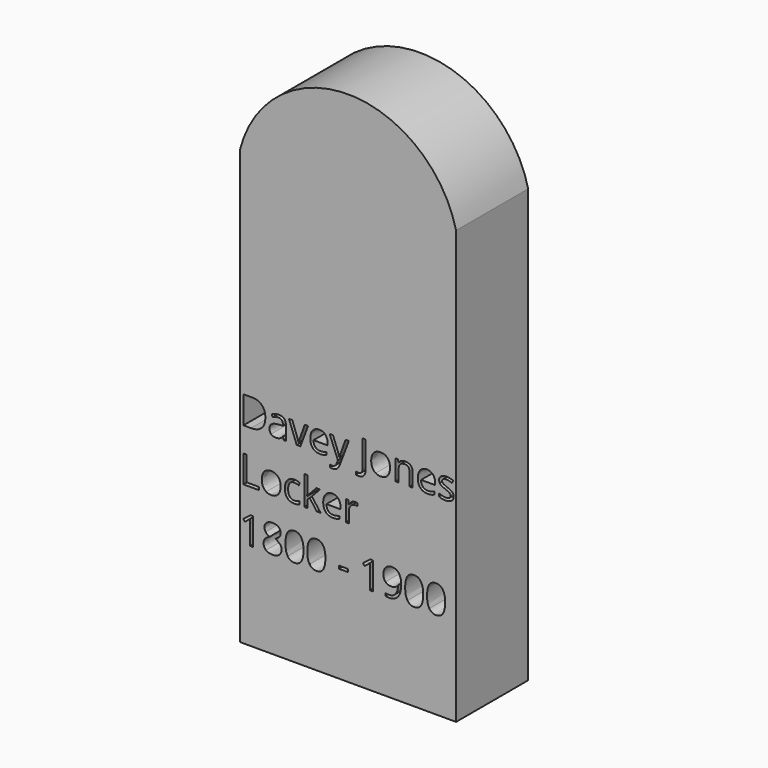
from build123d import *

# Parameters (mm, degrees)
F0_W     = 12.9239648405
F0_H     = 4.0018795953
F1_DEPTH = 127


with BuildPart() as f1:
    # F0 (on Front) → F1 (new body)
    with BuildSketch(Plane.XZ):
        with BuildLine():
            Line((-39.4293889403, 317.6073561937), (-39.4293889403, -291.9926438063))
            Line((-39.4293889403, -291.9926438063), (265.3706110597, -291.9926438063))
            Line((265.3706110597, -291.9926438063), (265.3706110597, 317.6073561937))
            ThreePointArc((265.3706110597, 317.6073561937), (112.9706110597, 436.9978931719), (-39.4293889403, 317.6073561937))
        make_face()
        with BuildLine():
            Line((-20.6079173278, -129.7050005513), (-20.6079173278, -168.1988697536))
            Line((-20.6079173278, -168.1988697536), (-24.870972223, -168.1988697536))
            Line((-24.870972223, -168.1988697536), (-24.870972223, -140.7670382538))
            add(Edge.make_bspline(
                [(-24.870972223, -140.7670382538), (-24.870972223, -137.3380593163), (-24.6603469811, -134.2882058142)],
                knots=[0, 0, 0, 1, 1, 1], degree=2))
            add(Edge.make_bspline(
                [(-24.6603469811, -134.2882058142), (-25.20797261, -134.8442564527), (-25.8946108984, -135.4466446444)],
                knots=[0, 0, 0, 1, 1, 1], degree=2))
            add(Edge.make_bspline(
                [(-25.8946108984, -135.4466446444), (-26.5812491869, -136.0490328361), (-32.1586055913, -140.5816880409)],
                knots=[0, 0, 0, 1, 1, 1], degree=2))
            Line((-32.1586055913, -140.5816880409), (-34.4754832518, -137.5823845969))
            Line((-34.4754832518, -137.5823845969), (-24.2896465555, -129.7050005513))
            Line((-24.2896465555, -129.7050005513), (-20.6079173278, -129.7050005513))
        make_face(mode=Mode.SUBTRACT)
        with BuildLine():
            add(Edge.make_bspline(
                [(-1.5084203959, -131.6427527764), (1.5835581546, -129.1573749225), (6.773364114, -129.1573749225)],
                knots=[0, 0, 0, 1, 1, 1], degree=2))
            add(Edge.make_bspline(
                [(6.773364114, -129.1573749225), (12.0389951605, -129.1573749225), (15.1183361965, -131.6048402329)],
                knots=[0, 0, 0, 1, 1, 1], degree=2))
            add(Edge.make_bspline(
                [(15.1183361965, -131.6048402329), (18.1976772325, -134.0523055433), (18.1976772325, -138.3659104966)],
                knots=[0, 0, 0, 1, 1, 1], degree=2))
            add(Edge.make_bspline(
                [(18.1976772325, -138.3659104966), (18.1976772325, -141.2135637665), (16.4368502105, -143.555716456)],
                knots=[0, 0, 0, 1, 1, 1], degree=2))
            add(Edge.make_bspline(
                [(16.4368502105, -143.555716456), (14.6760231886, -145.8978691455), (10.8005187384, -147.8187713512)],
                knots=[0, 0, 0, 1, 1, 1], degree=2))
            add(Edge.make_bspline(
                [(10.8005187384, -147.8187713512), (15.4848241173, -150.0598239246), (17.460488886, -152.5199267496)],
                knots=[0, 0, 0, 1, 1, 1], degree=2))
            add(Edge.make_bspline(
                [(17.460488886, -152.5199267496), (19.4361536546, -154.9800295745), (19.4361536546, -158.2236582991)],
                knots=[0, 0, 0, 1, 1, 1], degree=2))
            add(Edge.make_bspline(
                [(19.4361536546, -158.2236582991), (19.4361536546, -163.0090637942), (16.0914248139, -165.8693545786)],
                knots=[0, 0, 0, 1, 1, 1], degree=2))
            add(Edge.make_bspline(
                [(16.0914248139, -165.8693545786), (12.7466959731, -168.7296453631), (6.9334392978, -168.7296453631)],
                knots=[0, 0, 0, 1, 1, 1], degree=2))
            add(Edge.make_bspline(
                [(6.9334392978, -168.7296453631), (0.7747572258, -168.7296453631), (-2.5446965859, -166.0294297624)],
                knots=[0, 0, 0, 1, 1, 1], degree=2))
            add(Edge.make_bspline(
                [(-2.5446965859, -166.0294297624), (-5.8641503976, -163.3292141618), (-5.8641503976, -158.3753084732)],
                knots=[0, 0, 0, 1, 1, 1], degree=2))
            add(Edge.make_bspline(
                [(-5.8641503976, -158.3753084732), (-5.8641503976, -151.7701008885), (2.1901588511, -148.0799466511)],
                knots=[0, 0, 0, 1, 1, 1], degree=2))
            add(Edge.make_bspline(
                [(2.1901588511, -148.0799466511), (-1.4410203185, -146.0326693003), (-3.0207096325, -143.6483915624)],
                knots=[0, 0, 0, 1, 1, 1], degree=2))
            add(Edge.make_bspline(
                [(-3.0207096325, -143.6483915624), (-4.6003989464, -141.2641138246), (-4.6003989464, -138.3153604385)],
                knots=[0, 0, 0, 1, 1, 1], degree=2))
            add(Edge.make_bspline(
                [(-4.6003989464, -138.3153604385), (-4.6003989464, -134.1281306304), (-1.5084203959, -131.6427527764)],
                knots=[0, 0, 0, 1, 1, 1], degree=2))
        make_face(mode=Mode.SUBTRACT)
        with BuildLine():
            add(Edge.make_bspline(
                [(47.1207354447, -134.1828931932), (50.372789179, -139.2673865317), (50.372789179, -148.8971725896)],
                knots=[0, 0, 0, 1, 1, 1], degree=2))
            add(Edge.make_bspline(
                [(50.372789179, -148.8971725896), (50.372789179, -158.8808090537), (47.2260480656, -163.8052272084)],
                knots=[0, 0, 0, 1, 1, 1], degree=2))
            add(Edge.make_bspline(
                [(47.2260480656, -163.8052272084), (44.0793069522, -168.7296453631), (37.6004745126, -168.7296453631)],
                knots=[0, 0, 0, 1, 1, 1], degree=2))
            add(Edge.make_bspline(
                [(37.6004745126, -168.7296453631), (31.3912423826, -168.7296453631), (28.1518261628, -163.687277073)],
                knots=[0, 0, 0, 1, 1, 1], degree=2))
            add(Edge.make_bspline(
                [(28.1518261628, -163.687277073), (24.912409943, -158.6449087828), (24.912409943, -148.8971725896)],
                knots=[0, 0, 0, 1, 1, 1], degree=2))
            add(Edge.make_bspline(
                [(24.912409943, -148.8971725896), (24.912409943, -138.846136048), (28.0465135418, -133.9722679514)],
                knots=[0, 0, 0, 1, 1, 1], degree=2))
            add(Edge.make_bspline(
                [(28.0465135418, -133.9722679514), (31.1806171407, -129.0983998548), (37.6004745126, -129.0983998548)],
                knots=[0, 0, 0, 1, 1, 1], degree=2))
            add(Edge.make_bspline(
                [(37.6004745126, -129.0983998548), (43.8686817103, -129.0983998548), (47.1207354447, -134.1828931932)],
                knots=[0, 0, 0, 1, 1, 1], degree=2))
        make_face(mode=Mode.SUBTRACT)
        with BuildLine():
            add(Edge.make_bspline(
                [(77.9478458432, -134.1828931932), (81.1998995775, -139.2673865317), (81.1998995775, -148.8971725896)],
                knots=[0, 0, 0, 1, 1, 1], degree=2))
            add(Edge.make_bspline(
                [(81.1998995775, -148.8971725896), (81.1998995775, -158.8808090537), (78.0531584642, -163.8052272084)],
                knots=[0, 0, 0, 1, 1, 1], degree=2))
            add(Edge.make_bspline(
                [(78.0531584642, -163.8052272084), (74.9064173508, -168.7296453631), (68.4275849112, -168.7296453631)],
                knots=[0, 0, 0, 1, 1, 1], degree=2))
            add(Edge.make_bspline(
                [(68.4275849112, -168.7296453631), (62.2183527812, -168.7296453631), (58.9789365614, -163.687277073)],
                knots=[0, 0, 0, 1, 1, 1], degree=2))
            add(Edge.make_bspline(
                [(58.9789365614, -163.687277073), (55.7395203415, -158.6449087828), (55.7395203415, -148.8971725896)],
                knots=[0, 0, 0, 1, 1, 1], degree=2))
            add(Edge.make_bspline(
                [(55.7395203415, -148.8971725896), (55.7395203415, -138.846136048), (58.8736239404, -133.9722679514)],
                knots=[0, 0, 0, 1, 1, 1], degree=2))
            add(Edge.make_bspline(
                [(58.8736239404, -133.9722679514), (62.0077275393, -129.0983998548), (68.4275849112, -129.0983998548)],
                knots=[0, 0, 0, 1, 1, 1], degree=2))
            add(Edge.make_bspline(
                [(68.4275849112, -129.0983998548), (74.6957921089, -129.0983998548), (77.9478458432, -134.1828931932)],
                knots=[0, 0, 0, 1, 1, 1], degree=2))
        make_face(mode=Mode.SUBTRACT)
        with Locations((106.5676037071, -153.7457656572)):
            Rectangle(F0_W, F0_H, mode=Mode.SUBTRACT)
        Polygon((-12.6799832242, -94.8675855477), (-34.1384828648, -94.8675855477), (-34.1384828648, -56.3737163454), (-29.6648027277, -56.3737163454), (-29.6648027277, -90.8151558943), (-12.6799832242, -90.8151558943), align=None, mode=Mode.SUBTRACT)
        with BuildLine():
            add(Edge.make_bspline(
                [(14.5285855193, -69.5125189326), (18.0965771164, -73.5438860618), (18.0965771164, -80.4102689465)],
                knots=[0, 0, 0, 1, 1, 1], degree=2))
            add(Edge.make_bspline(
                [(18.0965771164, -80.4102689465), (18.0965771164, -87.4704270536), (14.5454355386, -91.4343941054)],
                knots=[0, 0, 0, 1, 1, 1], degree=2))
            add(Edge.make_bspline(
                [(14.5454355386, -91.4343941054), (10.9942939609, -95.3983611572), (4.7260867631, -95.3983611572)],
                knots=[0, 0, 0, 1, 1, 1], degree=2))
            add(Edge.make_bspline(
                [(4.7260867631, -95.3983611572), (0.8505823129, -95.3983611572), (-2.1487211312, -93.5785590675)],
                knots=[0, 0, 0, 1, 1, 1], degree=2))
            add(Edge.make_bspline(
                [(-2.1487211312, -93.5785590675), (-5.1480245753, -91.7587569779), (-6.7824764521, -88.3634780791)],
                knots=[0, 0, 0, 1, 1, 1], degree=2))
            add(Edge.make_bspline(
                [(-6.7824764521, -88.3634780791), (-8.4169283289, -84.9681991803), (-8.4169283289, -80.4102689465)],
                knots=[0, 0, 0, 1, 1, 1], degree=2))
            add(Edge.make_bspline(
                [(-8.4169283289, -80.4102689465), (-8.4169283289, -73.358535849), (-4.8868492753, -69.4198438262)],
                knots=[0, 0, 0, 1, 1, 1], degree=2))
            add(Edge.make_bspline(
                [(-4.8868492753, -69.4198438262), (-1.3567702218, -65.4811518035), (4.911436976, -65.4811518035)],
                knots=[0, 0, 0, 1, 1, 1], degree=2))
            add(Edge.make_bspline(
                [(4.911436976, -65.4811518035), (10.9605939222, -65.4811518035), (14.5285855193, -69.5125189326)],
                knots=[0, 0, 0, 1, 1, 1], degree=2))
        make_face(mode=Mode.SUBTRACT)
        with BuildLine():
            add(Edge.make_bspline(
                [(44.5848075327, -93.8902844255), (41.6950292143, -95.3983611572), (37.2971741643, -95.3983611572)],
                knots=[0, 0, 0, 1, 1, 1], degree=2))
            add(Edge.make_bspline(
                [(37.2971741643, -95.3983611572), (31.0289669666, -95.3983611572), (27.5915630194, -91.5397067263)],
                knots=[0, 0, 0, 1, 1, 1], degree=2))
            add(Edge.make_bspline(
                [(27.5915630194, -91.5397067263), (24.1541590723, -87.6810522955), (24.1541590723, -80.6208941883)],
                knots=[0, 0, 0, 1, 1, 1], degree=2))
            add(Edge.make_bspline(
                [(24.1541590723, -80.6208941883), (24.1541590723, -73.383810878), (27.6463255823, -69.4324813407)],
                knots=[0, 0, 0, 1, 1, 1], degree=2))
            add(Edge.make_bspline(
                [(27.6463255823, -69.4324813407), (31.1384920923, -65.4811518035), (37.5836244932, -65.4811518035)],
                knots=[0, 0, 0, 1, 1, 1], degree=2))
            add(Edge.make_bspline(
                [(37.5836244932, -65.4811518035), (39.6646018828, -65.4811518035), (41.7455792724, -65.931889821)],
                knots=[0, 0, 0, 1, 1, 1], degree=2))
            add(Edge.make_bspline(
                [(41.7455792724, -65.931889821), (43.826556662, -66.3826278386), (45.0060580164, -66.9892285352)],
                knots=[0, 0, 0, 1, 1, 1], degree=2))
            Line((45.0060580164, -66.9892285352), (43.6664814782, -70.6962327919))
            add(Edge.make_bspline(
                [(43.6664814782, -70.6962327919), (42.2173798142, -70.1149071244), (40.5071028503, -69.735781689)],
                knots=[0, 0, 0, 1, 1, 1], degree=2))
            add(Edge.make_bspline(
                [(40.5071028503, -69.735781689), (38.7968258864, -69.3566562537), (37.4825243772, -69.3566562537)],
                knots=[0, 0, 0, 1, 1, 1], degree=2))
            add(Edge.make_bspline(
                [(37.4825243772, -69.3566562537), (28.6868142771, -69.3566562537), (28.6868142771, -80.5703441303)],
                knots=[0, 0, 0, 1, 1, 1], degree=2))
            add(Edge.make_bspline(
                [(28.6868142771, -80.5703441303), (28.6868142771, -85.8865252348), (30.8309792392, -88.7299659999)],
                knots=[0, 0, 0, 1, 1, 1], degree=2))
            add(Edge.make_bspline(
                [(30.8309792392, -88.7299659999), (32.9751442014, -91.573406765), (37.1876490385, -91.573406765)],
                knots=[0, 0, 0, 1, 1, 1], degree=2))
            add(Edge.make_bspline(
                [(37.1876490385, -91.573406765), (40.7935531792, -91.573406765), (44.5848075327, -90.0232049849)],
                knots=[0, 0, 0, 1, 1, 1], degree=2))
            Line((44.5848075327, -90.0232049849), (44.5848075327, -93.8902844255))
        make_face(mode=Mode.SUBTRACT)
        with BuildLine():
            add(Edge.make_bspline(
                [(-8.3874407951, 11.9825996477), (-3.4124725823, 7.007631435), (-3.4124725823, -1.9228788199)],
                knots=[0, 0, 0, 1, 1, 1], degree=2))
            add(Edge.make_bspline(
                [(-3.4124725823, -1.9228788199), (-3.4124725823, -11.4515647616), (-8.5854285224, -16.4939330517)],
                knots=[0, 0, 0, 1, 1, 1], degree=2))
            add(Edge.make_bspline(
                [(-8.5854285224, -16.4939330517), (-13.7583844625, -21.5363013418), (-23.472420617, -21.5363013418)],
                knots=[0, 0, 0, 1, 1, 1], degree=2))
            Line((-23.472420617, -21.5363013418), (-34.1384828648, -21.5363013418))
            Line((-34.1384828648, -21.5363013418), (-34.1384828648, 16.9575678604))
            Line((-34.1384828648, 16.9575678604), (-22.3434693207, 16.9575678604))
            add(Edge.make_bspline(
                [(-22.3434693207, 16.9575678604), (-13.3624090078, 16.9575678604), (-8.3874407951, 11.9825996477)],
                knots=[0, 0, 0, 1, 1, 1], degree=2))
        make_face(mode=Mode.SUBTRACT)
        with BuildLine():
            Line((25.5021606202, -21.5363013418), (22.2585318955, -21.5363013418))
            Line((22.2585318955, -21.5363013418), (21.3907558991, -17.4248966207))
            Line((21.3907558991, -17.4248966207), (21.1801306572, -17.4248966207))
            add(Edge.make_bspline(
                [(21.1801306572, -17.4248966207), (19.0233281806, -20.1377497359), (16.8791632184, -21.1024133436)],
                knots=[0, 0, 0, 1, 1, 1], degree=2))
            add(Edge.make_bspline(
                [(16.8791632184, -21.1024133436), (14.7349982563, -22.0670769513), (11.5166445607, -22.0670769513)],
                knots=[0, 0, 0, 1, 1, 1], degree=2))
            add(Edge.make_bspline(
                [(11.5166445607, -22.0670769513), (7.2283146364, -22.0670769513), (4.7934868405, -19.851299407)],
                knots=[0, 0, 0, 1, 1, 1], degree=2))
            add(Edge.make_bspline(
                [(4.7934868405, -19.851299407), (2.3586590446, -17.6355218626), (2.3586590446, -13.5578171802)],
                knots=[0, 0, 0, 1, 1, 1], degree=2))
            add(Edge.make_bspline(
                [(2.3586590446, -13.5578171802), (2.3586590446, -4.8210821479), (16.3357500944, -4.3998316641)],
                knots=[0, 0, 0, 1, 1, 1], degree=2))
            Line((16.3357500944, -4.3998316641), (21.2306807153, -4.2397564803))
            Line((21.2306807153, -4.2397564803), (21.2306807153, -2.4452294197))
            add(Edge.make_bspline(
                [(21.2306807153, -2.4452294197), (21.2306807153, 0.9500494791), (19.7731540416, 2.5676513366)],
                knots=[0, 0, 0, 1, 1, 1], degree=2))
            add(Edge.make_bspline(
                [(19.7731540416, 2.5676513366), (18.3156273679, 4.1852531941), (15.0972736723, 4.1852531941)],
                knots=[0, 0, 0, 1, 1, 1], degree=2))
            add(Edge.make_bspline(
                [(15.0972736723, 4.1852531941), (11.4913695317, 4.1852531941), (6.9418643075, 1.9779006594)],
                knots=[0, 0, 0, 1, 1, 1], degree=2))
            Line((6.9418643075, 1.9779006594), (5.5938627596, 5.3226295001))
            add(Edge.make_bspline(
                [(5.5938627596, 5.3226295001), (7.7253902072, 6.4768558255), (10.265530624, 7.1340065801)],
                knots=[0, 0, 0, 1, 1, 1], degree=2))
            add(Edge.make_bspline(
                [(10.265530624, 7.1340065801), (12.8056710409, 7.7911573347), (15.3668739819, 7.7911573347)],
                knots=[0, 0, 0, 1, 1, 1], degree=2))
            add(Edge.make_bspline(
                [(15.3668739819, 7.7911573347), (20.5229799026, 7.7911573347), (23.0125702614, 5.5037672081)],
                knots=[0, 0, 0, 1, 1, 1], degree=2))
            add(Edge.make_bspline(
                [(23.0125702614, 5.5037672081), (25.5021606202, 3.2163770815), (25.5021606202, -1.8386287231)],
                knots=[0, 0, 0, 1, 1, 1], degree=2))
            Line((25.5021606202, -1.8386287231), (25.5021606202, -21.5363013418))
        make_face(mode=Mode.SUBTRACT)
        with BuildLine():
            Line((55.545745119, -80.0985435885), (55.7563703609, -80.0985435885))
            add(Edge.make_bspline(
                [(55.7563703609, -80.0985435885), (56.8853216573, -78.4893667407), (59.2021993177, -75.8860387513)],
                knots=[0, 0, 0, 1, 1, 1], degree=2))
            Line((59.2021993177, -75.8860387513), (68.5202600176, -66.0119274129))
            Line((68.5202600176, -66.0119274129), (73.710065977, -66.0119274129))
            Line((73.710065977, -66.0119274129), (62.016152549, -78.3040165279))
            Line((62.016152549, -78.3040165279), (74.5272919154, -94.8675855477))
            Line((74.5272919154, -94.8675855477), (69.2363858399, -94.8675855477))
            Line((69.2363858399, -94.8675855477), (59.0421241339, -81.2274948849))
            Line((59.0421241339, -81.2274948849), (55.7563703609, -84.0751481548))
            Line((55.7563703609, -84.0751481548), (55.7563703609, -94.8675855477))
            Line((55.7563703609, -94.8675855477), (51.4343403979, -94.8675855477))
            Line((51.4343403979, -94.8675855477), (51.4343403979, -53.8967635012))
            Line((51.4343403979, -53.8967635012), (55.7563703609, -53.8967635012))
            Line((55.7563703609, -53.8967635012), (55.7563703609, -75.6248634514))
            add(Edge.make_bspline(
                [(55.7563703609, -75.6248634514), (55.7563703609, -77.0655401057), (55.545745119, -80.0985435885)],
                knots=[0, 0, 0, 1, 1, 1], degree=2))
        make_face(mode=Mode.SUBTRACT)
        with BuildLine():
            add(Edge.make_bspline(
                [(96.9125426203, -94.9602606541), (94.8484152501, -95.3983611572), (91.924936893, -95.3983611572)],
                knots=[0, 0, 0, 1, 1, 1], degree=2))
            add(Edge.make_bspline(
                [(91.924936893, -95.3983611572), (85.5303545502, -95.3983611572), (81.8275627983, -91.497581678)],
                knots=[0, 0, 0, 1, 1, 1], degree=2))
            add(Edge.make_bspline(
                [(81.8275627983, -91.497581678), (78.1247710464, -87.5968021987), (78.1247710464, -80.679869256)],
                knots=[0, 0, 0, 1, 1, 1], degree=2))
            add(Edge.make_bspline(
                [(78.1247710464, -80.679869256), (78.1247710464, -73.695536236), (81.5621749935, -69.5883440197)],
                knots=[0, 0, 0, 1, 1, 1], degree=2))
            add(Edge.make_bspline(
                [(81.5621749935, -69.5883440197), (84.9995789407, -65.4811518035), (90.7959855967, -65.4811518035)],
                knots=[0, 0, 0, 1, 1, 1], degree=2))
            add(Edge.make_bspline(
                [(90.7959855967, -65.4811518035), (96.2132668173, -65.4811518035), (99.3726454452, -69.0491434006)],
                knots=[0, 0, 0, 1, 1, 1], degree=2))
            add(Edge.make_bspline(
                [(99.3726454452, -69.0491434006), (102.5320240731, -72.6171349977), (102.5320240731, -78.4640917117)],
                knots=[0, 0, 0, 1, 1, 1], degree=2))
            Line((102.5320240731, -78.4640917117), (102.5320240731, -81.2274948849))
            Line((102.5320240731, -81.2274948849), (82.6574262512, -81.2274948849))
            add(Edge.make_bspline(
                [(82.6574262512, -81.2274948849), (82.792226406, -86.3077757185), (85.2270542019, -88.9405912418)],
                knots=[0, 0, 0, 1, 1, 1], degree=2))
            add(Edge.make_bspline(
                [(85.2270542019, -88.9405912418), (87.6618819978, -91.573406765), (92.0850120769, -91.573406765)],
                knots=[0, 0, 0, 1, 1, 1], degree=2))
            add(Edge.make_bspline(
                [(92.0850120769, -91.573406765), (96.7440424268, -91.573406765), (101.293547651, -89.6272295302)],
                knots=[0, 0, 0, 1, 1, 1], degree=2))
            Line((101.293547651, -89.6272295302), (101.293547651, -93.5280090095))
            add(Edge.make_bspline(
                [(101.293547651, -93.5280090095), (98.9766699905, -94.5221601511), (96.9125426203, -94.9602606541)],
                knots=[0, 0, 0, 1, 1, 1], degree=2))
        make_face(mode=Mode.SUBTRACT)
        with BuildLine():
            Line((45.9243840709, -21.5363013418), (40.8188282082, -21.5363013418))
            Line((40.8188282082, -21.5363013418), (29.8663156315, 7.3193567929))
            Line((29.8663156315, 7.3193567929), (34.5506210105, 7.3193567929))
            Line((34.5506210105, 7.3193567929), (40.7682781502, -9.7918378557))
            add(Edge.make_bspline(
                [(40.7682781502, -9.7918378557), (42.8745305688, -15.7988697536), (43.2452309944, -17.5849718046)],
                knots=[0, 0, 0, 1, 1, 1], degree=2))
            Line((43.2452309944, -17.5849718046), (43.4558562363, -17.5849718046))
            add(Edge.make_bspline(
                [(43.4558562363, -17.5849718046), (43.7423065652, -16.1948452083), (45.2840833356, -11.8096276728)],
                knots=[0, 0, 0, 1, 1, 1], degree=2))
            add(Edge.make_bspline(
                [(45.2840833356, -11.8096276728), (46.825860106, -7.4244101372), (52.1925912686, 7.3193567929)],
                knots=[0, 0, 0, 1, 1, 1], degree=2))
            Line((52.1925912686, 7.3193567929), (56.8768966476, 7.3193567929))
            Line((56.8768966476, 7.3193567929), (45.9243840709, -21.5363013418))
        make_face(mode=Mode.SUBTRACT)
        with BuildLine():
            add(Edge.make_bspline(
                [(78.6892466946, -21.6289764483), (76.6251193244, -22.0670769513), (73.7016409673, -22.0670769513)],
                knots=[0, 0, 0, 1, 1, 1], degree=2))
            add(Edge.make_bspline(
                [(73.7016409673, -22.0670769513), (67.3070586245, -22.0670769513), (63.6042668726, -18.1662974721)],
                knots=[0, 0, 0, 1, 1, 1], degree=2))
            add(Edge.make_bspline(
                [(63.6042668726, -18.1662974721), (59.9014751207, -14.2655179928), (59.9014751207, -7.3485850502)],
                knots=[0, 0, 0, 1, 1, 1], degree=2))
            add(Edge.make_bspline(
                [(59.9014751207, -7.3485850502), (59.9014751207, -0.3642520301), (63.3388790678, 3.7429401862)],
                knots=[0, 0, 0, 1, 1, 1], degree=2))
            add(Edge.make_bspline(
                [(63.3388790678, 3.7429401862), (66.776283015, 7.8501324024), (72.572689671, 7.8501324024)],
                knots=[0, 0, 0, 1, 1, 1], degree=2))
            add(Edge.make_bspline(
                [(72.572689671, 7.8501324024), (77.9899708916, 7.8501324024), (81.1493495195, 4.2821408053)],
                knots=[0, 0, 0, 1, 1, 1], degree=2))
            add(Edge.make_bspline(
                [(81.1493495195, 4.2821408053), (84.3087281474, 0.7141492082), (84.3087281474, -5.1328075058)],
                knots=[0, 0, 0, 1, 1, 1], degree=2))
            Line((84.3087281474, -5.1328075058), (84.3087281474, -7.896210679))
            Line((84.3087281474, -7.896210679), (64.4341303255, -7.896210679))
            add(Edge.make_bspline(
                [(64.4341303255, -7.896210679), (64.5689304803, -12.9764915127), (67.0037582762, -15.6093070359)],
                knots=[0, 0, 0, 1, 1, 1], degree=2))
            add(Edge.make_bspline(
                [(67.0037582762, -15.6093070359), (69.4385860721, -18.2421225592), (73.8617161512, -18.2421225592)],
                knots=[0, 0, 0, 1, 1, 1], degree=2))
            add(Edge.make_bspline(
                [(73.8617161512, -18.2421225592), (78.5207465011, -18.2421225592), (83.0702517253, -16.2959453244)],
                knots=[0, 0, 0, 1, 1, 1], degree=2))
            Line((83.0702517253, -16.2959453244), (83.0702517253, -20.1967248036))
            add(Edge.make_bspline(
                [(83.0702517253, -20.1967248036), (80.7533740648, -21.1908759452), (78.6892466946, -21.6289764483)],
                knots=[0, 0, 0, 1, 1, 1], degree=2))
        make_face(mode=Mode.SUBTRACT)
        with BuildLine():
            Line((98.8250198164, -21.6963765257), (87.1816564464, 7.3193567929))
            Line((87.1816564464, 7.3193567929), (91.874386835, 7.3193567929))
            Line((91.874386835, 7.3193567929), (98.1931440908, -9.1346871011))
            add(Edge.make_bspline(
                [(98.1931440908, -9.1346871011), (100.2656964707, -14.7710185733), (100.7711970512, -17.2732464466)],
                knots=[0, 0, 0, 1, 1, 1], degree=2))
            Line((100.7711970512, -17.2732464466), (100.981822293, -17.2732464466))
            add(Edge.make_bspline(
                [(100.981822293, -17.2732464466), (101.31882268, -15.9252448987), (102.4140739377, -12.6731911644)],
                knots=[0, 0, 0, 1, 1, 1], degree=2))
            add(Edge.make_bspline(
                [(102.4140739377, -12.6731911644), (103.5093251953, -9.4211374301), (109.5669071512, 7.3193567929)],
                knots=[0, 0, 0, 1, 1, 1], degree=2))
            Line((109.5669071512, 7.3193567929), (114.2512125302, 7.3193567929))
            Line((114.2512125302, 7.3193567929), (101.8495982895, -25.5381809372))
            add(Edge.make_bspline(
                [(101.8495982895, -25.5381809372), (100.0045211708, -30.407836529), (97.5444183459, -32.450901375)],
                knots=[0, 0, 0, 1, 1, 1], degree=2))
            add(Edge.make_bspline(
                [(97.5444183459, -32.450901375), (95.0843155209, -34.4939662211), (91.5036864093, -34.4939662211)],
                knots=[0, 0, 0, 1, 1, 1], degree=2))
            add(Edge.make_bspline(
                [(91.5036864093, -34.4939662211), (89.4985341068, -34.4939662211), (87.552356872, -34.0390156986)],
                knots=[0, 0, 0, 1, 1, 1], degree=2))
            Line((87.552356872, -34.0390156986), (87.552356872, -30.5426366838))
            add(Edge.make_bspline(
                [(87.552356872, -30.5426366838), (89.001458536, -30.8543620417), (90.787560587, -30.8543620417)],
                knots=[0, 0, 0, 1, 1, 1], degree=2))
            add(Edge.make_bspline(
                [(90.787560587, -30.8543620417), (95.2949407628, -30.8543620417), (97.2158429686, -25.7993562371)],
                knots=[0, 0, 0, 1, 1, 1], degree=2))
            Line((97.2158429686, -25.7993562371), (98.8250198164, -21.6963765257))
        make_face(mode=Mode.SUBTRACT)
        with BuildLine():
            Line((148.0692013632, -129.7050005513), (148.0692013632, -168.1988697536))
            Line((148.0692013632, -168.1988697536), (143.8061464679, -168.1988697536))
            Line((143.8061464679, -168.1988697536), (143.8061464679, -140.7670382538))
            add(Edge.make_bspline(
                [(143.8061464679, -140.7670382538), (143.8061464679, -137.3380593163), (144.0167717098, -134.2882058142)],
                knots=[0, 0, 0, 1, 1, 1], degree=2))
            add(Edge.make_bspline(
                [(144.0167717098, -134.2882058142), (143.4691460809, -134.8442564527), (142.7825077925, -135.4466446444)],
                knots=[0, 0, 0, 1, 1, 1], degree=2))
            add(Edge.make_bspline(
                [(142.7825077925, -135.4466446444), (142.095869504, -136.0490328361), (136.5185130996, -140.5816880409)],
                knots=[0, 0, 0, 1, 1, 1], degree=2))
            Line((136.5185130996, -140.5816880409), (134.2016354391, -137.5823845969))
            Line((134.2016354391, -137.5823845969), (144.3874721355, -129.7050005513))
            Line((144.3874721355, -129.7050005513), (148.0692013632, -129.7050005513))
        make_face(mode=Mode.SUBTRACT)
        with BuildLine():
            add(Edge.make_bspline(
                [(186.4324829155, -137.0389714729), (188.0121722294, -140.8934133989), (188.0121722294, -146.1337694164)],
                knots=[0, 0, 0, 1, 1, 1], degree=2))
            add(Edge.make_bspline(
                [(188.0121722294, -146.1337694164), (188.0121722294, -168.7296453631), (170.5302771551, -168.7296453631)],
                knots=[0, 0, 0, 1, 1, 1], degree=2))
            add(Edge.make_bspline(
                [(170.5302771551, -168.7296453631), (167.4719986433, -168.7296453631), (165.6858965923, -168.1988697536)],
                knots=[0, 0, 0, 1, 1, 1], degree=2))
            Line((165.6858965923, -168.1988697536), (165.6858965923, -164.4328904291))
            add(Edge.make_bspline(
                [(165.6858965923, -164.4328904291), (167.7921490109, -165.1153162128), (170.4713020874, -165.1153162128)],
                knots=[0, 0, 0, 1, 1, 1], degree=2))
            add(Edge.make_bspline(
                [(170.4713020874, -165.1153162128), (176.7900593432, -165.1153162128), (180.0168380484, -161.2061117238)],
                knots=[0, 0, 0, 1, 1, 1], degree=2))
            add(Edge.make_bspline(
                [(180.0168380484, -161.2061117238), (183.2436167537, -157.2969072349), (183.5300670827, -149.2173229572)],
                knots=[0, 0, 0, 1, 1, 1], degree=2))
            Line((183.5300670827, -149.2173229572), (183.2183417247, -149.2173229572))
            add(Edge.make_bspline(
                [(183.2183417247, -149.2173229572), (181.7692400607, -151.3994004629), (179.3723248084, -152.5452017786)],
                knots=[0, 0, 0, 1, 1, 1], degree=2))
            add(Edge.make_bspline(
                [(179.3723248084, -152.5452017786), (176.975409556, -153.6910030943), (173.9761061119, -153.6910030943)],
                knots=[0, 0, 0, 1, 1, 1], degree=2))
            add(Edge.make_bspline(
                [(173.9761061119, -153.6910030943), (168.8705502492, -153.6910030943), (165.8670343003, -150.6369370873)],
                knots=[0, 0, 0, 1, 1, 1], degree=2))
            add(Edge.make_bspline(
                [(165.8670343003, -150.6369370873), (162.8635183514, -147.5828710804), (162.8635183514, -142.106614792)],
                knots=[0, 0, 0, 1, 1, 1], degree=2))
            add(Edge.make_bspline(
                [(162.8635183514, -142.106614792), (162.8635183514, -136.1080079038), (166.2208847066, -132.6326914132)],
                knots=[0, 0, 0, 1, 1, 1], degree=2))
            add(Edge.make_bspline(
                [(166.2208847066, -132.6326914132), (169.5782510619, -129.1573749225), (175.0545073502, -129.1573749225)],
                knots=[0, 0, 0, 1, 1, 1], degree=2))
            add(Edge.make_bspline(
                [(175.0545073502, -129.1573749225), (178.9805618585, -129.1573749225), (181.91667773, -131.1709522347)],
                knots=[0, 0, 0, 1, 1, 1], degree=2))
            add(Edge.make_bspline(
                [(181.91667773, -131.1709522347), (184.8527936015, -133.1845295468), (186.4324829155, -137.0389714729)],
                knots=[0, 0, 0, 1, 1, 1], degree=2))
        make_face(mode=Mode.SUBTRACT)
        with BuildLine():
            add(Edge.make_bspline(
                [(215.7978541356, -134.1828931932), (219.0499078699, -139.2673865317), (219.0499078699, -148.8971725896)],
                knots=[0, 0, 0, 1, 1, 1], degree=2))
            add(Edge.make_bspline(
                [(219.0499078699, -148.8971725896), (219.0499078699, -158.8808090537), (215.9031667565, -163.8052272084)],
                knots=[0, 0, 0, 1, 1, 1], degree=2))
            add(Edge.make_bspline(
                [(215.9031667565, -163.8052272084), (212.7564256431, -168.7296453631), (206.2775932035, -168.7296453631)],
                knots=[0, 0, 0, 1, 1, 1], degree=2))
            add(Edge.make_bspline(
                [(206.2775932035, -168.7296453631), (200.0683610735, -168.7296453631), (196.8289448537, -163.687277073)],
                knots=[0, 0, 0, 1, 1, 1], degree=2))
            add(Edge.make_bspline(
                [(196.8289448537, -163.687277073), (193.5895286339, -158.6449087828), (193.5895286339, -148.8971725896)],
                knots=[0, 0, 0, 1, 1, 1], degree=2))
            add(Edge.make_bspline(
                [(193.5895286339, -148.8971725896), (193.5895286339, -138.846136048), (196.7236322328, -133.9722679514)],
                knots=[0, 0, 0, 1, 1, 1], degree=2))
            add(Edge.make_bspline(
                [(196.7236322328, -133.9722679514), (199.8577358316, -129.0983998548), (206.2775932035, -129.0983998548)],
                knots=[0, 0, 0, 1, 1, 1], degree=2))
            add(Edge.make_bspline(
                [(206.2775932035, -129.0983998548), (212.5458004013, -129.0983998548), (215.7978541356, -134.1828931932)],
                knots=[0, 0, 0, 1, 1, 1], degree=2))
        make_face(mode=Mode.SUBTRACT)
        with BuildLine():
            add(Edge.make_bspline(
                [(246.6249645342, -134.1828931932), (249.8770182685, -139.2673865317), (249.8770182685, -148.8971725896)],
                knots=[0, 0, 0, 1, 1, 1], degree=2))
            add(Edge.make_bspline(
                [(249.8770182685, -148.8971725896), (249.8770182685, -158.8808090537), (246.7302771551, -163.8052272084)],
                knots=[0, 0, 0, 1, 1, 1], degree=2))
            add(Edge.make_bspline(
                [(246.7302771551, -163.8052272084), (243.5835360417, -168.7296453631), (237.1047036021, -168.7296453631)],
                knots=[0, 0, 0, 1, 1, 1], degree=2))
            add(Edge.make_bspline(
                [(237.1047036021, -168.7296453631), (230.8954714721, -168.7296453631), (227.6560552523, -163.687277073)],
                knots=[0, 0, 0, 1, 1, 1], degree=2))
            add(Edge.make_bspline(
                [(227.6560552523, -163.687277073), (224.4166390325, -158.6449087828), (224.4166390325, -148.8971725896)],
                knots=[0, 0, 0, 1, 1, 1], degree=2))
            add(Edge.make_bspline(
                [(224.4166390325, -148.8971725896), (224.4166390325, -138.846136048), (227.5507426313, -133.9722679514)],
                knots=[0, 0, 0, 1, 1, 1], degree=2))
            add(Edge.make_bspline(
                [(227.5507426313, -133.9722679514), (230.6848462302, -129.0983998548), (237.1047036021, -129.0983998548)],
                knots=[0, 0, 0, 1, 1, 1], degree=2))
            add(Edge.make_bspline(
                [(237.1047036021, -129.0983998548), (243.3729107998, -129.0983998548), (246.6249645342, -134.1828931932)],
                knots=[0, 0, 0, 1, 1, 1], degree=2))
        make_face(mode=Mode.SUBTRACT)
        with BuildLine():
            add(Edge.make_bspline(
                [(118.1772670384, -67.0102910594), (120.4435946408, -65.4811518035), (123.156447756, -65.4811518035)],
                knots=[0, 0, 0, 1, 1, 1], degree=2))
            add(Edge.make_bspline(
                [(123.156447756, -65.4811518035), (125.0773499618, -65.4811518035), (126.6022767128, -65.8013021711)],
                knots=[0, 0, 0, 1, 1, 1], degree=2))
            Line((126.6022767128, -65.8013021711), (125.9956760163, -69.8537318245))
            add(Edge.make_bspline(
                [(125.9956760163, -69.8537318245), (124.2095739653, -69.4577563698), (122.8362973884, -69.4577563698)],
                knots=[0, 0, 0, 1, 1, 1], degree=2))
            add(Edge.make_bspline(
                [(122.8362973884, -69.4577563698), (119.3314933638, -69.4577563698), (116.8461155099, -72.3011971349)],
                knots=[0, 0, 0, 1, 1, 1], degree=2))
            add(Edge.make_bspline(
                [(116.8461155099, -72.3011971349), (114.3607376559, -75.1446379), (114.3607376559, -79.3824177662)],
                knots=[0, 0, 0, 1, 1, 1], degree=2))
            Line((114.3607376559, -79.3824177662), (114.3607376559, -94.8675855477))
            Line((114.3607376559, -94.8675855477), (109.9881576349, -94.8675855477))
            Line((109.9881576349, -94.8675855477), (109.9881576349, -66.0119274129))
            Line((109.9881576349, -66.0119274129), (113.5940617756, -66.0119274129))
            Line((113.5940617756, -66.0119274129), (114.099562356, -71.3533835465))
            Line((114.099562356, -71.3533835465), (114.3101875979, -71.3533835465))
            add(Edge.make_bspline(
                [(114.3101875979, -71.3533835465), (115.910939436, -68.5394303153), (118.1772670384, -67.0102910594)],
                knots=[0, 0, 0, 1, 1, 1], degree=2))
        make_face(mode=Mode.SUBTRACT)
        with BuildLine():
            add(Edge.make_bspline(
                [(135.2631866581, -28.9208223214), (132.7356837558, -31.6715879801), (127.9924033091, -31.6715879801)],
                knots=[0, 0, 0, 1, 1, 1], degree=2))
            add(Edge.make_bspline(
                [(127.9924033091, -31.6715879801), (125.5238754745, -31.6715879801), (124.1000488395, -30.9638871675)],
                knots=[0, 0, 0, 1, 1, 1], degree=2))
            Line((124.1000488395, -30.9638871675), (124.1000488395, -27.147357785))
            add(Edge.make_bspline(
                [(124.1000488395, -27.147357785), (125.9704009872, -27.6697083848), (127.9924033091, -27.6697083848)],
                knots=[0, 0, 0, 1, 1, 1], degree=2))
            add(Edge.make_bspline(
                [(127.9924033091, -27.6697083848), (130.6041563082, -27.6697083848), (131.9605828657, -26.0900190709)],
                knots=[0, 0, 0, 1, 1, 1], degree=2))
            add(Edge.make_bspline(
                [(131.9605828657, -26.0900190709), (133.3170094233, -24.5103297569), (133.3170094233, -21.5363013418)],
                knots=[0, 0, 0, 1, 1, 1], degree=2))
            Line((133.3170094233, -21.5363013418), (133.3170094233, 16.9575678604))
            Line((133.3170094233, 16.9575678604), (137.7906895604, 16.9575678604))
            Line((137.7906895604, 16.9575678604), (137.7906895604, -21.1656009162))
            add(Edge.make_bspline(
                [(137.7906895604, -21.1656009162), (137.7906895604, -26.1700566628), (135.2631866581, -28.9208223214)],
                knots=[0, 0, 0, 1, 1, 1], degree=2))
        make_face(mode=Mode.SUBTRACT)
        with BuildLine():
            add(Edge.make_bspline(
                [(168.6809875316, 3.8187652732), (172.2489791287, -0.212601856), (172.2489791287, -7.0789847406)],
                knots=[0, 0, 0, 1, 1, 1], degree=2))
            add(Edge.make_bspline(
                [(172.2489791287, -7.0789847406), (172.2489791287, -14.1391428477), (168.6978375509, -18.1031098995)],
                knots=[0, 0, 0, 1, 1, 1], degree=2))
            add(Edge.make_bspline(
                [(168.6978375509, -18.1031098995), (165.1466959731, -22.0670769513), (158.8784887754, -22.0670769513)],
                knots=[0, 0, 0, 1, 1, 1], degree=2))
            add(Edge.make_bspline(
                [(158.8784887754, -22.0670769513), (155.0029843252, -22.0670769513), (152.0036808811, -20.2472748617)],
                knots=[0, 0, 0, 1, 1, 1], degree=2))
            add(Edge.make_bspline(
                [(152.0036808811, -20.2472748617), (149.004377437, -18.427472772), (147.3699255602, -15.0321938732)],
                knots=[0, 0, 0, 1, 1, 1], degree=2))
            add(Edge.make_bspline(
                [(147.3699255602, -15.0321938732), (145.7354736834, -11.6369149744), (145.7354736834, -7.0789847406)],
                knots=[0, 0, 0, 1, 1, 1], degree=2))
            add(Edge.make_bspline(
                [(145.7354736834, -7.0789847406), (145.7354736834, -0.0272516431), (149.2655527369, 3.9114403796)],
                knots=[0, 0, 0, 1, 1, 1], degree=2))
            add(Edge.make_bspline(
                [(149.2655527369, 3.9114403796), (152.7956317905, 7.8501324024), (159.0638389882, 7.8501324024)],
                knots=[0, 0, 0, 1, 1, 1], degree=2))
            add(Edge.make_bspline(
                [(159.0638389882, 7.8501324024), (165.1129959345, 7.8501324024), (168.6809875316, 3.8187652732)],
                knots=[0, 0, 0, 1, 1, 1], degree=2))
        make_face(mode=Mode.SUBTRACT)
        with BuildLine():
            Line((204.0365406301, -21.5363013418), (199.6639606091, -21.5363013418))
            Line((199.6639606091, -21.5363013418), (199.6639606091, -2.8664799034))
            add(Edge.make_bspline(
                [(199.6639606091, -2.8664799034), (199.6639606091, 0.6551741405), (198.0589962661, 2.3949386383)],
                knots=[0, 0, 0, 1, 1, 1], degree=2))
            add(Edge.make_bspline(
                [(198.0589962661, 2.3949386383), (196.4540319232, 4.134703136), (193.0250529857, 4.134703136)],
                knots=[0, 0, 0, 1, 1, 1], degree=2))
            add(Edge.make_bspline(
                [(193.0250529857, 4.134703136), (188.5008227906, 4.134703136), (186.394570372, 1.6872378256)],
                knots=[0, 0, 0, 1, 1, 1], degree=2))
            add(Edge.make_bspline(
                [(186.394570372, 1.6872378256), (184.2883179534, -0.7602274848), (184.2883179534, -6.396558957)],
                knots=[0, 0, 0, 1, 1, 1], degree=2))
            Line((184.2883179534, -6.396558957), (184.2883179534, -21.5363013418))
            Line((184.2883179534, -21.5363013418), (179.9157379324, -21.5363013418))
            Line((179.9157379324, -21.5363013418), (179.9157379324, 7.3193567929))
            Line((179.9157379324, 7.3193567929), (183.4710920149, 7.3193567929))
            Line((183.4710920149, 7.3193567929), (184.1787928276, 3.3680272556))
            Line((184.1787928276, 3.3680272556), (184.3894180695, 3.3680272556))
            add(Edge.make_bspline(
                [(184.3894180695, 3.3680272556), (185.7374196174, 5.4995547033), (188.1596098987, 6.6748435528)],
                knots=[0, 0, 0, 1, 1, 1], degree=2))
            add(Edge.make_bspline(
                [(188.1596098987, 6.6748435528), (190.5818001801, 7.8501324024), (193.5558285952, 7.8501324024)],
                knots=[0, 0, 0, 1, 1, 1], degree=2))
            add(Edge.make_bspline(
                [(193.5558285952, 7.8501324024), (198.7709095836, 7.8501324024), (201.4037251069, 5.3352670146)],
                knots=[0, 0, 0, 1, 1, 1], degree=2))
            add(Edge.make_bspline(
                [(201.4037251069, 5.3352670146), (204.0365406301, 2.8204016268), (204.0365406301, -2.7148297293)],
                knots=[0, 0, 0, 1, 1, 1], degree=2))
            Line((204.0365406301, -2.7148297293), (204.0365406301, -21.5363013418))
        make_face(mode=Mode.SUBTRACT)
        with BuildLine():
            add(Edge.make_bspline(
                [(230.1877706594, -21.6289764483), (228.1236432892, -22.0670769513), (225.2001649322, -22.0670769513)],
                knots=[0, 0, 0, 1, 1, 1], degree=2))
            add(Edge.make_bspline(
                [(225.2001649322, -22.0670769513), (218.8055825893, -22.0670769513), (215.1027908374, -18.1662974721)],
                knots=[0, 0, 0, 1, 1, 1], degree=2))
            add(Edge.make_bspline(
                [(215.1027908374, -18.1662974721), (211.3999990855, -14.2655179928), (211.3999990855, -7.3485850502)],
                knots=[0, 0, 0, 1, 1, 1], degree=2))
            add(Edge.make_bspline(
                [(211.3999990855, -7.3485850502), (211.3999990855, -0.3642520301), (214.8374030327, 3.7429401862)],
                knots=[0, 0, 0, 1, 1, 1], degree=2))
            add(Edge.make_bspline(
                [(214.8374030327, 3.7429401862), (218.2748069798, 7.8501324024), (224.0712136358, 7.8501324024)],
                knots=[0, 0, 0, 1, 1, 1], degree=2))
            add(Edge.make_bspline(
                [(224.0712136358, 7.8501324024), (229.4884948564, 7.8501324024), (232.6478734843, 4.2821408053)],
                knots=[0, 0, 0, 1, 1, 1], degree=2))
            add(Edge.make_bspline(
                [(232.6478734843, 4.2821408053), (235.8072521122, 0.7141492082), (235.8072521122, -5.1328075058)],
                knots=[0, 0, 0, 1, 1, 1], degree=2))
            Line((235.8072521122, -5.1328075058), (235.8072521122, -7.896210679))
            Line((235.8072521122, -7.896210679), (215.9326542904, -7.896210679))
            add(Edge.make_bspline(
                [(215.9326542904, -7.896210679), (216.0674544451, -12.9764915127), (218.502282241, -15.6093070359)],
                knots=[0, 0, 0, 1, 1, 1], degree=2))
            add(Edge.make_bspline(
                [(218.502282241, -15.6093070359), (220.9371100369, -18.2421225592), (225.360240116, -18.2421225592)],
                knots=[0, 0, 0, 1, 1, 1], degree=2))
            add(Edge.make_bspline(
                [(225.360240116, -18.2421225592), (230.0192704659, -18.2421225592), (234.5687756901, -16.2959453244)],
                knots=[0, 0, 0, 1, 1, 1], degree=2))
            Line((234.5687756901, -16.2959453244), (234.5687756901, -20.1967248036))
            add(Edge.make_bspline(
                [(234.5687756901, -20.1967248036), (232.2518980296, -21.1908759452), (230.1877706594, -21.6289764483)],
                knots=[0, 0, 0, 1, 1, 1], degree=2))
        make_face(mode=Mode.SUBTRACT)
        with BuildLine():
            add(Edge.make_bspline(
                [(260.0712799745, -8.8987868303), (261.8742320448, -10.794414007), (261.8742320448, -13.667342306)],
                knots=[0, 0, 0, 1, 1, 1], degree=2))
            add(Edge.make_bspline(
                [(261.8742320448, -13.667342306), (261.8742320448, -17.6944969303), (258.8749286007, -19.8807869408)],
                knots=[0, 0, 0, 1, 1, 1], degree=2))
            add(Edge.make_bspline(
                [(258.8749286007, -19.8807869408), (255.8756251566, -22.0670769513), (250.4499189263, -22.0670769513)],
                knots=[0, 0, 0, 1, 1, 1], degree=2))
            add(Edge.make_bspline(
                [(250.4499189263, -22.0670769513), (244.7124873381, -22.0670769513), (241.5025586521, -20.2472748617)],
                knots=[0, 0, 0, 1, 1, 1], degree=2))
            Line((241.5025586521, -20.2472748617), (241.5025586521, -16.1948452083))
            add(Edge.make_bspline(
                [(241.5025586521, -16.1948452083), (243.5835360417, -17.2479714176), (245.9636012747, -17.8503596093)],
                knots=[0, 0, 0, 1, 1, 1], degree=2))
            add(Edge.make_bspline(
                [(245.9636012747, -17.8503596093), (248.3436665077, -18.452747801), (250.5594440521, -18.452747801)],
                knots=[0, 0, 0, 1, 1, 1], degree=2))
            add(Edge.make_bspline(
                [(250.5594440521, -18.452747801), (253.9799979799, -18.452747801), (255.8208625937, -17.3617090482)],
                knots=[0, 0, 0, 1, 1, 1], degree=2))
            add(Edge.make_bspline(
                [(255.8208625937, -17.3617090482), (257.6617272076, -16.2706702954), (257.6617272076, -14.029617722)],
                knots=[0, 0, 0, 1, 1, 1], degree=2))
            add(Edge.make_bspline(
                [(257.6617272076, -14.029617722), (257.6617272076, -12.3446157871), (256.2042005339, -11.1482644133)],
                knots=[0, 0, 0, 1, 1, 1], degree=2))
            add(Edge.make_bspline(
                [(256.2042005339, -11.1482644133), (254.7466738603, -9.9519130396), (250.5004689844, -8.3174611627)],
                knots=[0, 0, 0, 1, 1, 1], degree=2))
            add(Edge.make_bspline(
                [(250.5004689844, -8.3174611627), (246.47331436, -6.8178094407), (244.7756749106, -5.697283154)],
                knots=[0, 0, 0, 1, 1, 1], degree=2))
            add(Edge.make_bspline(
                [(244.7756749106, -5.697283154), (243.0780354612, -4.5767568673), (242.2481720083, -3.1571427372)],
                knots=[0, 0, 0, 1, 1, 1], degree=2))
            add(Edge.make_bspline(
                [(242.2481720083, -3.1571427372), (241.4183085554, -1.737528607), (241.4183085554, 0.2339236568)],
                knots=[0, 0, 0, 1, 1, 1], degree=2))
            add(Edge.make_bspline(
                [(241.4183085554, 0.2339236568), (241.4183085554, 3.7640027103), (244.2912368543, 5.8070675564)],
                knots=[0, 0, 0, 1, 1, 1], degree=2))
            add(Edge.make_bspline(
                [(244.2912368543, 5.8070675564), (247.1641651533, 7.8501324024), (252.1601958902, 7.8501324024)],
                knots=[0, 0, 0, 1, 1, 1], degree=2))
            add(Edge.make_bspline(
                [(252.1601958902, 7.8501324024), (256.8192262402, 7.8501324024), (261.2760563579, 5.9545052257)],
                knots=[0, 0, 0, 1, 1, 1], degree=2))
            Line((261.2760563579, 5.9545052257), (259.7174295682, 2.3991511431))
            add(Edge.make_bspline(
                [(259.7174295682, 2.3991511431), (255.3785495858, 4.1852531941), (251.8484705323, 4.1852531941)],
                knots=[0, 0, 0, 1, 1, 1], degree=2))
            add(Edge.make_bspline(
                [(251.8484705323, 4.1852531941), (248.7396419624, 4.1852531941), (247.1599526485, 3.2121645767)],
                knots=[0, 0, 0, 1, 1, 1], degree=2))
            add(Edge.make_bspline(
                [(247.1599526485, 3.2121645767), (245.5802633345, 2.2390759593), (245.5802633345, 0.5287989954)],
                knots=[0, 0, 0, 1, 1, 1], degree=2))
            add(Edge.make_bspline(
                [(245.5802633345, 0.5287989954), (245.5802633345, -0.6338523397), (246.1742265166, -1.4468657733)],
                knots=[0, 0, 0, 1, 1, 1], degree=2))
            add(Edge.make_bspline(
                [(246.1742265166, -1.4468657733), (246.7681896986, -2.2598792068), (248.0824912078, -2.9970675534)],
                knots=[0, 0, 0, 1, 1, 1], degree=2))
            add(Edge.make_bspline(
                [(248.0824912078, -2.9970675534), (249.396792717, -3.7342558999), (253.1374970125, -5.1328075058)],
                knots=[0, 0, 0, 1, 1, 1], degree=2))
            add(Edge.make_bspline(
                [(253.1374970125, -5.1328075058), (258.2683279042, -7.0031596535), (260.0712799745, -8.8987868303)],
                knots=[0, 0, 0, 1, 1, 1], degree=2))
        make_face(mode=Mode.SUBTRACT)
    extrude(amount=F1_DEPTH)


solid = f1.part
